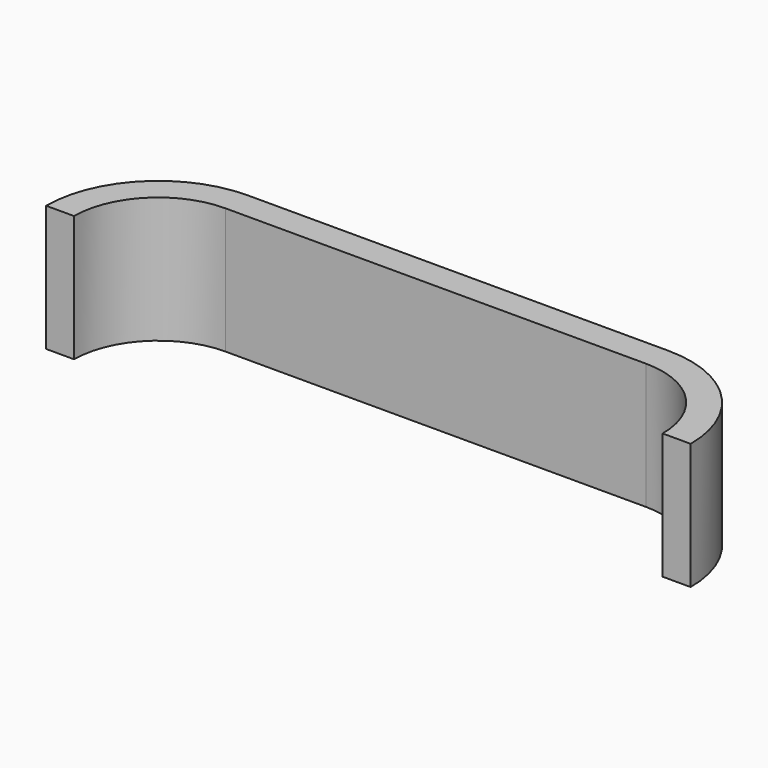
from build123d import *

# Parameters (mm, degrees)
F1_DEPTH = 4.5
F2_R     = 2.99999
F3_R     = 3.99999


# Not quite as in the source:
# - a fillet or chamfer is up to 0.001 mm smaller than in the source, because OpenCascade refuses the exact size


with BuildPart() as f1:
    # F0 (on Top) → F1 (new body)
    with BuildSketch(Plane.XY):
        Polygon((10.5, 3), (10.5, 0), (11.5, 0), (11.5, 4), (-11.5, 4), (-11.5, 0), (-10.5, 0), (-10.5, 3), align=None)
    extrude(amount=F1_DEPTH)

    # F2 (radius 3 in the source; OpenCascade refuses exactly that, so slightly less here)
    f2_edges = [f1.edges().sort_by_distance(p)[0] for p in [
        (10.5, 3, 2.25),
        (-10.5, 3, 2.25),
    ]]
    fillet(f2_edges, radius=F2_R)

    # F3 (radius 4 in the source; OpenCascade refuses exactly that, so slightly less here)
    f3_edges = [f1.edges().sort_by_distance(p)[0] for p in [
        (-11.5, 4, 2.25),
        (11.5, 4, 2.25),
    ]]
    fillet(f3_edges, radius=F3_R)


solid = f1.part
